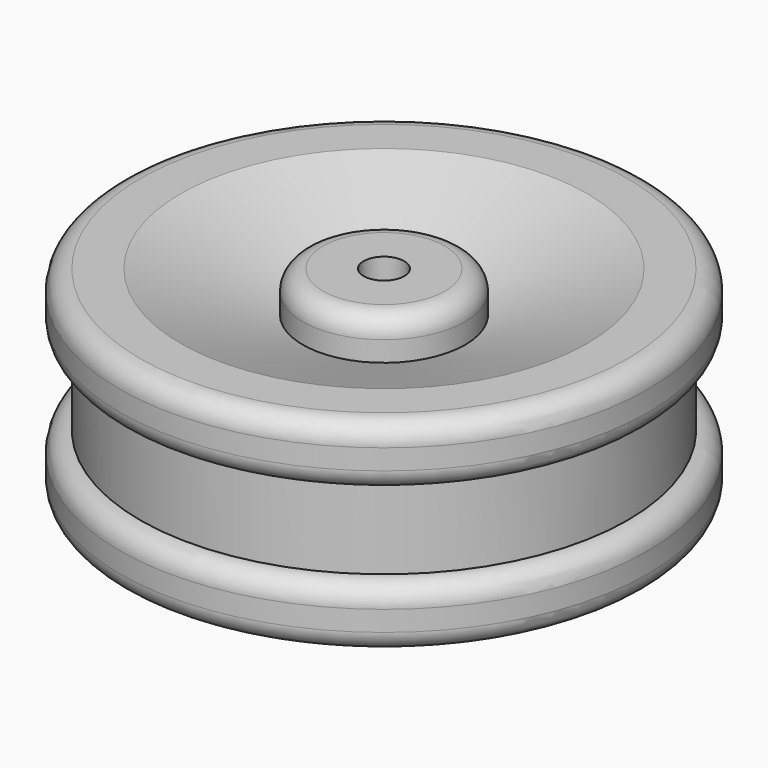
from build123d import *

# Parameters (mm, degrees)
F0_R      = 13
F0_R_2    = 1
F1_DEPTH  = 10
F4_R      = 10
F3_R      = 4
F8_R      = 10
F7_R      = 4
F11_R     = 4
F11_R_2   = 1
F12_DEPTH = 2
F14_R     = 13
F14_R_2   = 12
F15_DEPTH = 4
F16_R     = 0.99999


# Not quite as in the source:
# - a fillet or chamfer is up to 0.001 mm smaller than in the source, because OpenCascade refuses the exact size
# - a feature of the source that left no trace in its solid (it failed there, or was rolled back) is left out
# - a pattern or mirror of a feature is missing from the dataset's text; its kind, count and spacing are read off the source's solid


with BuildPart() as f1:
    # F0 (on Top) → F1 (new body)
    with BuildSketch(Plane.XY):
        Circle(F0_R)
        Circle(F0_R_2, mode=Mode.SUBTRACT)
    extrude(amount=F1_DEPTH)

    # F4 (on face) → F5 section 0
    with BuildSketch(Plane.XY.offset(10)):
        Circle(F4_R)
    # F3 (on offset) → F5 section 1
    with BuildSketch(Plane.XY.offset(8)):
        Circle(F3_R)
    loft(mode=Mode.SUBTRACT)

    # F8 (on face) → F9 section 0
    with BuildSketch(Plane.XY):
        Circle(F8_R)
    # F7 (on offset) → F9 section 1
    with BuildSketch(Plane.XY.offset(2)):
        Circle(F7_R)
    loft(mode=Mode.SUBTRACT)

    # F11 (on face) → F12 (join, through all)
    with BuildSketch(Plane.XY):
        Circle(F11_R)
        Circle(F11_R_2, mode=Mode.SUBTRACT)
    f12 = extrude(amount=F12_DEPTH)

    # F12_copies: F12 across plane
    add(f12.mirror(Plane.XY.offset(5)))

    # F14 (on offset) → F15 (cut)
    with BuildSketch(Plane.XY.offset(3)):
        Circle(F14_R)
        Circle(F14_R_2, mode=Mode.SUBTRACT)
    extrude(amount=F15_DEPTH, mode=Mode.SUBTRACT)

    # F16 (radius 1 in the source; OpenCascade refuses exactly that, so slightly less here)
    f16_edges = [f1.edges().sort_by_distance(p)[0] for p in [
        (-4, 0, 0),
        (-13, 0, 10),
        (-13, 0, 0),
        (-13, 0, 7),
        (-13, 0, 3),
        (-4, 0, 10),
    ]]
    fillet(f16_edges, radius=F16_R)


solid = f1.part
